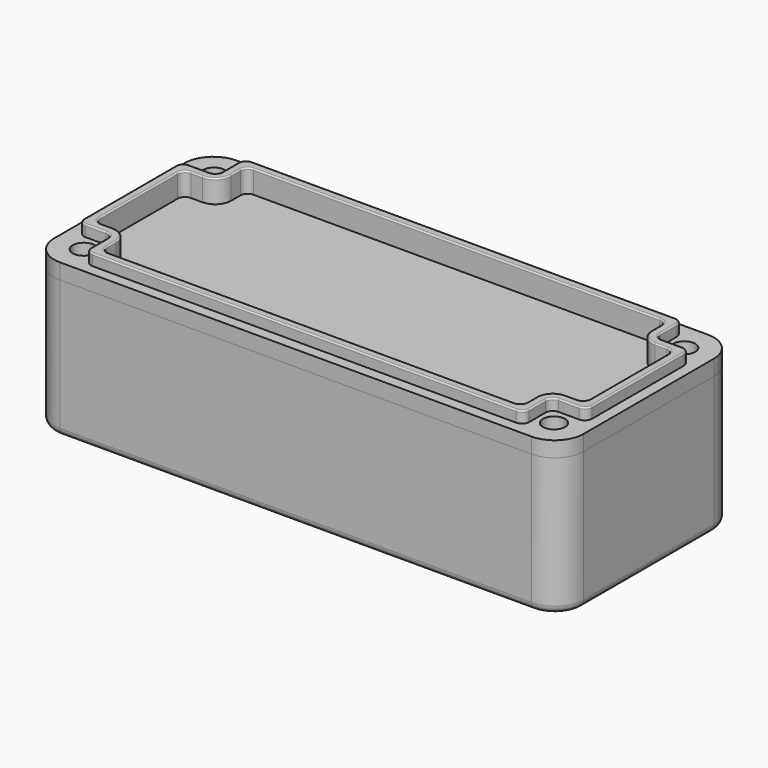
from build123d import *

# Parameters (mm, degrees)
F0_R     = 1.9431
F1_DEPTH = 26.924
F2_DEPTH = 25.4
F3_DEPTH = 3.9878
F4_DEPTH = 2.032
F5_DEPTH = 1.9812
F6_R     = 1.27
F7_SIZE  = 1.778
F8_SIZE  = 1.778
F9_R     = 0.254
F10_R    = 1.27


with BuildPart() as f1:
    # F0 (on Top) → F1 (new body)
    with BuildSketch(Plane.XY):
        with BuildLine():
            ThreePointArc((46.482, 14.2875), (44.9941024484, 17.8796024484), (41.402, 19.3675))
            Line((41.402, 19.3675), (38.4556, 19.3675))
            Line((38.4556, 19.3675), (-41.402, 19.3675))
            ThreePointArc((-41.402, 19.3675), (-44.9941024484, 17.8796024484), (-46.482, 14.2875))
            Line((-46.482, 14.2875), (-46.482, -11.3411))
            Line((-46.482, -11.3411), (-46.482, -14.2875))
            ThreePointArc((-46.482, -14.2875), (-44.9941024484, -17.8796024484), (-41.402, -19.3675))
            Line((-41.402, -19.3675), (-38.4556, -19.3675))
            Line((-38.4556, -19.3675), (38.4556, -19.3675))
            Line((38.4556, -19.3675), (41.402, -19.3675))
            ThreePointArc((41.402, -19.3675), (44.9941024484, -17.8796024484), (46.482, -14.2875))
            Line((46.482, -14.2875), (46.482, -11.3411))
            Line((46.482, -11.3411), (46.482, 11.3411))
            Line((46.482, 11.3411), (46.482, 14.2875))
        make_face()
        with Locations((-41.275, -14.2875)):
            Circle(F0_R, mode=Mode.SUBTRACT)
        with Locations((41.275, -14.2875)):
            Circle(F0_R, mode=Mode.SUBTRACT)
        with Locations((-41.275, 14.2875)):
            Circle(F0_R, mode=Mode.SUBTRACT)
        with BuildLine():
            ThreePointArc((38.4556, -16.1925), (38.0836256121, -17.0905256121), (37.1856, -17.4625))
            Line((37.1856, -17.4625), (-37.1856, -17.4625))
            ThreePointArc((-37.1856, -17.4625), (-38.0836256121, -17.0905256121), (-38.4556, -16.1925))
            Line((-38.4556, -16.1925), (-38.4556, -12.6111))
            ThreePointArc((-38.4556, -12.6111), (-38.8275743879, -11.7130743879), (-39.7256, -11.3411))
            Line((-39.7256, -11.3411), (-43.307, -11.3411))
            ThreePointArc((-43.307, -11.3411), (-44.2050256121, -10.9691256121), (-44.577, -10.0711))
            Line((-44.577, -10.0711), (-44.577, 10.0711))
            ThreePointArc((-44.577, 10.0711), (-44.2050256121, 10.9691256121), (-43.307, 11.3411))
            Line((-43.307, 11.3411), (-39.7256, 11.3411))
            ThreePointArc((-39.7256, 11.3411), (-38.8275743879, 11.7130743879), (-38.4556, 12.6111))
            Line((-38.4556, 12.6111), (-38.4556, 16.1925))
            ThreePointArc((-38.4556, 16.1925), (-38.0836256121, 17.0905256121), (-37.1856, 17.4625))
            Line((-37.1856, 17.4625), (37.1856, 17.4625))
            ThreePointArc((37.1856, 17.4625), (38.0836256121, 17.0905256121), (38.4556, 16.1925))
            Line((38.4556, 16.1925), (38.4556, 12.6111))
            ThreePointArc((38.4556, 12.6111), (38.8275743879, 11.7130743879), (39.7256, 11.3411))
            Line((39.7256, 11.3411), (43.307, 11.3411))
            ThreePointArc((43.307, 11.3411), (44.2050256121, 10.9691256121), (44.577, 10.0711))
            Line((44.577, 10.0711), (44.577, -10.0711))
            ThreePointArc((44.577, -10.0711), (44.2050256121, -10.9691256121), (43.307, -11.3411))
            Line((43.307, -11.3411), (39.7256, -11.3411))
            ThreePointArc((39.7256, -11.3411), (38.8275743879, -11.7130743879), (38.4556, -12.6111))
            Line((38.4556, -12.6111), (38.4556, -16.1925))
        make_face(mode=Mode.SUBTRACT)
        with Locations((41.275, 14.2875)):
            Circle(F0_R, mode=Mode.SUBTRACT)
        with BuildLine():
            Line((-37.1856, -17.4625), (37.1856, -17.4625))
            ThreePointArc((37.1856, -17.4625), (38.0836256121, -17.0905256121), (38.4556, -16.1925))
            Line((38.4556, -16.1925), (38.4556, -12.6111))
            ThreePointArc((38.4556, -12.6111), (38.8275743879, -11.7130743879), (39.7256, -11.3411))
            Line((39.7256, -11.3411), (43.307, -11.3411))
            ThreePointArc((43.307, -11.3411), (44.2050256121, -10.9691256121), (44.577, -10.0711))
            Line((44.577, -10.0711), (44.577, 10.0711))
            ThreePointArc((44.577, 10.0711), (44.2050256121, 10.9691256121), (43.307, 11.3411))
            Line((43.307, 11.3411), (39.7256, 11.3411))
            ThreePointArc((39.7256, 11.3411), (38.8275743879, 11.7130743879), (38.4556, 12.6111))
            Line((38.4556, 12.6111), (38.4556, 16.1925))
            ThreePointArc((38.4556, 16.1925), (38.0836256121, 17.0905256121), (37.1856, 17.4625))
            Line((37.1856, 17.4625), (-37.1856, 17.4625))
            ThreePointArc((-37.1856, 17.4625), (-38.0836256121, 17.0905256121), (-38.4556, 16.1925))
            Line((-38.4556, 16.1925), (-38.4556, 12.6111))
            ThreePointArc((-38.4556, 12.6111), (-38.8275743879, 11.7130743879), (-39.7256, 11.3411))
            Line((-39.7256, 11.3411), (-43.307, 11.3411))
            ThreePointArc((-43.307, 11.3411), (-44.2050256121, 10.9691256121), (-44.577, 10.0711))
            Line((-44.577, 10.0711), (-44.577, -10.0711))
            ThreePointArc((-44.577, -10.0711), (-44.2050256121, -10.9691256121), (-43.307, -11.3411))
            Line((-43.307, -11.3411), (-39.7256, -11.3411))
            ThreePointArc((-39.7256, -11.3411), (-38.8275743879, -11.7130743879), (-38.4556, -12.6111))
            Line((-38.4556, -12.6111), (-38.4556, -16.1925))
            ThreePointArc((-38.4556, -16.1925), (-38.0836256121, -17.0905256121), (-37.1856, -17.4625))
        make_face()
        with BuildLine():
            Line((-35.6616, 15.9385), (35.6616, 15.9385))
            ThreePointArc((35.6616, 15.9385), (36.5596256121, 15.5665256121), (36.9316, 14.6685))
            Line((36.9316, 14.6685), (36.9316, 12.6111))
            ThreePointArc((36.9316, 12.6111), (37.7499436534, 10.6354436534), (39.7256, 9.8171))
            Line((39.7256, 9.8171), (41.783, 9.8171))
            ThreePointArc((41.783, 9.8171), (42.6810256121, 9.4451256121), (43.053, 8.5471))
            Line((43.053, 8.5471), (43.053, -8.5471))
            ThreePointArc((43.053, -8.5471), (42.6810256121, -9.4451256121), (41.783, -9.8171))
            Line((41.783, -9.8171), (39.7256, -9.8171))
            ThreePointArc((39.7256, -9.8171), (37.7499436534, -10.6354436534), (36.9316, -12.6111))
            Line((36.9316, -12.6111), (36.9316, -14.6685))
            ThreePointArc((36.9316, -14.6685), (36.5596256121, -15.5665256121), (35.6616, -15.9385))
            Line((35.6616, -15.9385), (-35.6616, -15.9385))
            ThreePointArc((-35.6616, -15.9385), (-36.5596256121, -15.5665256121), (-36.9316, -14.6685))
            Line((-36.9316, -14.6685), (-36.9316, -12.6111))
            ThreePointArc((-36.9316, -12.6111), (-37.7499436534, -10.6354436534), (-39.7256, -9.8171))
            Line((-39.7256, -9.8171), (-41.783, -9.8171))
            ThreePointArc((-41.783, -9.8171), (-42.6810256121, -9.4451256121), (-43.053, -8.5471))
            Line((-43.053, -8.5471), (-43.053, 8.5471))
            ThreePointArc((-43.053, 8.5471), (-42.6810256121, 9.4451256121), (-41.783, 9.8171))
            Line((-41.783, 9.8171), (-39.7256, 9.8171))
            ThreePointArc((-39.7256, 9.8171), (-37.7499436534, 10.6354436534), (-36.9316, 12.6111))
            Line((-36.9316, 12.6111), (-36.9316, 14.6685))
            ThreePointArc((-36.9316, 14.6685), (-36.5596256121, 15.5665256121), (-35.6616, 15.9385))
        make_face(mode=Mode.SUBTRACT)
        with Locations((41.275, 14.2875)):
            Circle(F0_R)
        with Locations((41.275, -14.2875)):
            Circle(F0_R)
        with Locations((-41.275, -14.2875)):
            Circle(F0_R)
        with Locations((-41.275, 14.2875)):
            Circle(F0_R)
        with BuildLine():
            ThreePointArc((36.9316, 14.6685), (36.5596256121, 15.5665256121), (35.6616, 15.9385))
            Line((35.6616, 15.9385), (-35.6616, 15.9385))
            ThreePointArc((-35.6616, 15.9385), (-36.5596256121, 15.5665256121), (-36.9316, 14.6685))
            Line((-36.9316, 14.6685), (-36.9316, 12.6111))
            ThreePointArc((-36.9316, 12.6111), (-37.7499436534, 10.6354436534), (-39.7256, 9.8171))
            Line((-39.7256, 9.8171), (-41.783, 9.8171))
            ThreePointArc((-41.783, 9.8171), (-42.6810256121, 9.4451256121), (-43.053, 8.5471))
            Line((-43.053, 8.5471), (-43.053, -8.5471))
            ThreePointArc((-43.053, -8.5471), (-42.6810256121, -9.4451256121), (-41.783, -9.8171))
            Line((-41.783, -9.8171), (-39.7256, -9.8171))
            ThreePointArc((-39.7256, -9.8171), (-37.7499436534, -10.6354436534), (-36.9316, -12.6111))
            Line((-36.9316, -12.6111), (-36.9316, -14.6685))
            ThreePointArc((-36.9316, -14.6685), (-36.5596256121, -15.5665256121), (-35.6616, -15.9385))
            Line((-35.6616, -15.9385), (35.6616, -15.9385))
            ThreePointArc((35.6616, -15.9385), (36.5596256121, -15.5665256121), (36.9316, -14.6685))
            Line((36.9316, -14.6685), (36.9316, -12.6111))
            ThreePointArc((36.9316, -12.6111), (37.7499436534, -10.6354436534), (39.7256, -9.8171))
            Line((39.7256, -9.8171), (41.783, -9.8171))
            ThreePointArc((41.783, -9.8171), (42.6810256121, -9.4451256121), (43.053, -8.5471))
            Line((43.053, -8.5471), (43.053, 8.5471))
            ThreePointArc((43.053, 8.5471), (42.6810256121, 9.4451256121), (41.783, 9.8171))
            Line((41.783, 9.8171), (39.7256, 9.8171))
            ThreePointArc((39.7256, 9.8171), (37.7499436534, 10.6354436534), (36.9316, 12.6111))
            Line((36.9316, 12.6111), (36.9316, 14.6685))
        make_face()
    extrude(amount=-F1_DEPTH)

    # F0 (on Top) → F2 (cut)
    with BuildSketch(Plane.XY):
        with Locations((-41.275, 14.2875)):
            Circle(F0_R)
        with Locations((-41.275, -14.2875)):
            Circle(F0_R)
        with BuildLine():
            Line((-37.1856, -17.4625), (37.1856, -17.4625))
            ThreePointArc((37.1856, -17.4625), (38.0836256121, -17.0905256121), (38.4556, -16.1925))
            Line((38.4556, -16.1925), (38.4556, -12.6111))
            ThreePointArc((38.4556, -12.6111), (38.8275743879, -11.7130743879), (39.7256, -11.3411))
            Line((39.7256, -11.3411), (43.307, -11.3411))
            ThreePointArc((43.307, -11.3411), (44.2050256121, -10.9691256121), (44.577, -10.0711))
            Line((44.577, -10.0711), (44.577, 10.0711))
            ThreePointArc((44.577, 10.0711), (44.2050256121, 10.9691256121), (43.307, 11.3411))
            Line((43.307, 11.3411), (39.7256, 11.3411))
            ThreePointArc((39.7256, 11.3411), (38.8275743879, 11.7130743879), (38.4556, 12.6111))
            Line((38.4556, 12.6111), (38.4556, 16.1925))
            ThreePointArc((38.4556, 16.1925), (38.0836256121, 17.0905256121), (37.1856, 17.4625))
            Line((37.1856, 17.4625), (-37.1856, 17.4625))
            ThreePointArc((-37.1856, 17.4625), (-38.0836256121, 17.0905256121), (-38.4556, 16.1925))
            Line((-38.4556, 16.1925), (-38.4556, 12.6111))
            ThreePointArc((-38.4556, 12.6111), (-38.8275743879, 11.7130743879), (-39.7256, 11.3411))
            Line((-39.7256, 11.3411), (-43.307, 11.3411))
            ThreePointArc((-43.307, 11.3411), (-44.2050256121, 10.9691256121), (-44.577, 10.0711))
            Line((-44.577, 10.0711), (-44.577, -10.0711))
            ThreePointArc((-44.577, -10.0711), (-44.2050256121, -10.9691256121), (-43.307, -11.3411))
            Line((-43.307, -11.3411), (-39.7256, -11.3411))
            ThreePointArc((-39.7256, -11.3411), (-38.8275743879, -11.7130743879), (-38.4556, -12.6111))
            Line((-38.4556, -12.6111), (-38.4556, -16.1925))
            ThreePointArc((-38.4556, -16.1925), (-38.0836256121, -17.0905256121), (-37.1856, -17.4625))
        make_face()
        with BuildLine():
            Line((-35.6616, 15.9385), (35.6616, 15.9385))
            ThreePointArc((35.6616, 15.9385), (36.5596256121, 15.5665256121), (36.9316, 14.6685))
            Line((36.9316, 14.6685), (36.9316, 12.6111))
            ThreePointArc((36.9316, 12.6111), (37.7499436534, 10.6354436534), (39.7256, 9.8171))
            Line((39.7256, 9.8171), (41.783, 9.8171))
            ThreePointArc((41.783, 9.8171), (42.6810256121, 9.4451256121), (43.053, 8.5471))
            Line((43.053, 8.5471), (43.053, -8.5471))
            ThreePointArc((43.053, -8.5471), (42.6810256121, -9.4451256121), (41.783, -9.8171))
            Line((41.783, -9.8171), (39.7256, -9.8171))
            ThreePointArc((39.7256, -9.8171), (37.7499436534, -10.6354436534), (36.9316, -12.6111))
            Line((36.9316, -12.6111), (36.9316, -14.6685))
            ThreePointArc((36.9316, -14.6685), (36.5596256121, -15.5665256121), (35.6616, -15.9385))
            Line((35.6616, -15.9385), (-35.6616, -15.9385))
            ThreePointArc((-35.6616, -15.9385), (-36.5596256121, -15.5665256121), (-36.9316, -14.6685))
            Line((-36.9316, -14.6685), (-36.9316, -12.6111))
            ThreePointArc((-36.9316, -12.6111), (-37.7499436534, -10.6354436534), (-39.7256, -9.8171))
            Line((-39.7256, -9.8171), (-41.783, -9.8171))
            ThreePointArc((-41.783, -9.8171), (-42.6810256121, -9.4451256121), (-43.053, -8.5471))
            Line((-43.053, -8.5471), (-43.053, 8.5471))
            ThreePointArc((-43.053, 8.5471), (-42.6810256121, 9.4451256121), (-41.783, 9.8171))
            Line((-41.783, 9.8171), (-39.7256, 9.8171))
            ThreePointArc((-39.7256, 9.8171), (-37.7499436534, 10.6354436534), (-36.9316, 12.6111))
            Line((-36.9316, 12.6111), (-36.9316, 14.6685))
            ThreePointArc((-36.9316, 14.6685), (-36.5596256121, 15.5665256121), (-35.6616, 15.9385))
        make_face(mode=Mode.SUBTRACT)
        with Locations((41.275, 14.2875)):
            Circle(F0_R)
        with Locations((41.275, -14.2875)):
            Circle(F0_R)
        with BuildLine():
            ThreePointArc((36.9316, 14.6685), (36.5596256121, 15.5665256121), (35.6616, 15.9385))
            Line((35.6616, 15.9385), (-35.6616, 15.9385))
            ThreePointArc((-35.6616, 15.9385), (-36.5596256121, 15.5665256121), (-36.9316, 14.6685))
            Line((-36.9316, 14.6685), (-36.9316, 12.6111))
            ThreePointArc((-36.9316, 12.6111), (-37.7499436534, 10.6354436534), (-39.7256, 9.8171))
            Line((-39.7256, 9.8171), (-41.783, 9.8171))
            ThreePointArc((-41.783, 9.8171), (-42.6810256121, 9.4451256121), (-43.053, 8.5471))
            Line((-43.053, 8.5471), (-43.053, -8.5471))
            ThreePointArc((-43.053, -8.5471), (-42.6810256121, -9.4451256121), (-41.783, -9.8171))
            Line((-41.783, -9.8171), (-39.7256, -9.8171))
            ThreePointArc((-39.7256, -9.8171), (-37.7499436534, -10.6354436534), (-36.9316, -12.6111))
            Line((-36.9316, -12.6111), (-36.9316, -14.6685))
            ThreePointArc((-36.9316, -14.6685), (-36.5596256121, -15.5665256121), (-35.6616, -15.9385))
            Line((-35.6616, -15.9385), (35.6616, -15.9385))
            ThreePointArc((35.6616, -15.9385), (36.5596256121, -15.5665256121), (36.9316, -14.6685))
            Line((36.9316, -14.6685), (36.9316, -12.6111))
            ThreePointArc((36.9316, -12.6111), (37.7499436534, -10.6354436534), (39.7256, -9.8171))
            Line((39.7256, -9.8171), (41.783, -9.8171))
            ThreePointArc((41.783, -9.8171), (42.6810256121, -9.4451256121), (43.053, -8.5471))
            Line((43.053, -8.5471), (43.053, 8.5471))
            ThreePointArc((43.053, 8.5471), (42.6810256121, 9.4451256121), (41.783, 9.8171))
            Line((41.783, 9.8171), (39.7256, 9.8171))
            ThreePointArc((39.7256, 9.8171), (37.7499436534, 10.6354436534), (36.9316, 12.6111))
            Line((36.9316, 12.6111), (36.9316, 14.6685))
        make_face()
    extrude(amount=-F2_DEPTH, mode=Mode.SUBTRACT)

    # F10
    f10_edges = [f1.edges().sort_by_distance(p)[0] for p in [
        (0, 19.3675, -26.924),
        (44.994102, -17.879602, -26.924),
        (0, -19.3675, -26.924),
        (46.482, 0, -26.924),
        (44.994102, 17.879602, -26.924),
        (-44.994102, 17.879602, -26.924),
        (-46.482, 0, -26.924),
        (-44.994102, -17.879602, -26.924),
    ]]
    fillet(f10_edges, radius=F10_R)


with BuildPart() as f3:
    # F0 (on Top) → F3 (new body)
    with BuildSketch(Plane.XY):
        with BuildLine():
            ThreePointArc((46.482, 14.2875), (44.9941024484, 17.8796024484), (41.402, 19.3675))
            Line((41.402, 19.3675), (38.4556, 19.3675))
            Line((38.4556, 19.3675), (-41.402, 19.3675))
            ThreePointArc((-41.402, 19.3675), (-44.9941024484, 17.8796024484), (-46.482, 14.2875))
            Line((-46.482, 14.2875), (-46.482, -11.3411))
            Line((-46.482, -11.3411), (-46.482, -14.2875))
            ThreePointArc((-46.482, -14.2875), (-44.9941024484, -17.8796024484), (-41.402, -19.3675))
            Line((-41.402, -19.3675), (-38.4556, -19.3675))
            Line((-38.4556, -19.3675), (38.4556, -19.3675))
            Line((38.4556, -19.3675), (41.402, -19.3675))
            ThreePointArc((41.402, -19.3675), (44.9941024484, -17.8796024484), (46.482, -14.2875))
            Line((46.482, -14.2875), (46.482, -11.3411))
            Line((46.482, -11.3411), (46.482, 11.3411))
            Line((46.482, 11.3411), (46.482, 14.2875))
        make_face()
        with Locations((-41.275, -14.2875)):
            Circle(F0_R, mode=Mode.SUBTRACT)
        with Locations((41.275, -14.2875)):
            Circle(F0_R, mode=Mode.SUBTRACT)
        with Locations((-41.275, 14.2875)):
            Circle(F0_R, mode=Mode.SUBTRACT)
        with BuildLine():
            ThreePointArc((38.4556, -16.1925), (38.0836256121, -17.0905256121), (37.1856, -17.4625))
            Line((37.1856, -17.4625), (-37.1856, -17.4625))
            ThreePointArc((-37.1856, -17.4625), (-38.0836256121, -17.0905256121), (-38.4556, -16.1925))
            Line((-38.4556, -16.1925), (-38.4556, -12.6111))
            ThreePointArc((-38.4556, -12.6111), (-38.8275743879, -11.7130743879), (-39.7256, -11.3411))
            Line((-39.7256, -11.3411), (-43.307, -11.3411))
            ThreePointArc((-43.307, -11.3411), (-44.2050256121, -10.9691256121), (-44.577, -10.0711))
            Line((-44.577, -10.0711), (-44.577, 10.0711))
            ThreePointArc((-44.577, 10.0711), (-44.2050256121, 10.9691256121), (-43.307, 11.3411))
            Line((-43.307, 11.3411), (-39.7256, 11.3411))
            ThreePointArc((-39.7256, 11.3411), (-38.8275743879, 11.7130743879), (-38.4556, 12.6111))
            Line((-38.4556, 12.6111), (-38.4556, 16.1925))
            ThreePointArc((-38.4556, 16.1925), (-38.0836256121, 17.0905256121), (-37.1856, 17.4625))
            Line((-37.1856, 17.4625), (37.1856, 17.4625))
            ThreePointArc((37.1856, 17.4625), (38.0836256121, 17.0905256121), (38.4556, 16.1925))
            Line((38.4556, 16.1925), (38.4556, 12.6111))
            ThreePointArc((38.4556, 12.6111), (38.8275743879, 11.7130743879), (39.7256, 11.3411))
            Line((39.7256, 11.3411), (43.307, 11.3411))
            ThreePointArc((43.307, 11.3411), (44.2050256121, 10.9691256121), (44.577, 10.0711))
            Line((44.577, 10.0711), (44.577, -10.0711))
            ThreePointArc((44.577, -10.0711), (44.2050256121, -10.9691256121), (43.307, -11.3411))
            Line((43.307, -11.3411), (39.7256, -11.3411))
            ThreePointArc((39.7256, -11.3411), (38.8275743879, -11.7130743879), (38.4556, -12.6111))
            Line((38.4556, -12.6111), (38.4556, -16.1925))
        make_face(mode=Mode.SUBTRACT)
        with Locations((41.275, 14.2875)):
            Circle(F0_R, mode=Mode.SUBTRACT)
        with BuildLine():
            Line((-37.1856, -17.4625), (37.1856, -17.4625))
            ThreePointArc((37.1856, -17.4625), (38.0836256121, -17.0905256121), (38.4556, -16.1925))
            Line((38.4556, -16.1925), (38.4556, -12.6111))
            ThreePointArc((38.4556, -12.6111), (38.8275743879, -11.7130743879), (39.7256, -11.3411))
            Line((39.7256, -11.3411), (43.307, -11.3411))
            ThreePointArc((43.307, -11.3411), (44.2050256121, -10.9691256121), (44.577, -10.0711))
            Line((44.577, -10.0711), (44.577, 10.0711))
            ThreePointArc((44.577, 10.0711), (44.2050256121, 10.9691256121), (43.307, 11.3411))
            Line((43.307, 11.3411), (39.7256, 11.3411))
            ThreePointArc((39.7256, 11.3411), (38.8275743879, 11.7130743879), (38.4556, 12.6111))
            Line((38.4556, 12.6111), (38.4556, 16.1925))
            ThreePointArc((38.4556, 16.1925), (38.0836256121, 17.0905256121), (37.1856, 17.4625))
            Line((37.1856, 17.4625), (-37.1856, 17.4625))
            ThreePointArc((-37.1856, 17.4625), (-38.0836256121, 17.0905256121), (-38.4556, 16.1925))
            Line((-38.4556, 16.1925), (-38.4556, 12.6111))
            ThreePointArc((-38.4556, 12.6111), (-38.8275743879, 11.7130743879), (-39.7256, 11.3411))
            Line((-39.7256, 11.3411), (-43.307, 11.3411))
            ThreePointArc((-43.307, 11.3411), (-44.2050256121, 10.9691256121), (-44.577, 10.0711))
            Line((-44.577, 10.0711), (-44.577, -10.0711))
            ThreePointArc((-44.577, -10.0711), (-44.2050256121, -10.9691256121), (-43.307, -11.3411))
            Line((-43.307, -11.3411), (-39.7256, -11.3411))
            ThreePointArc((-39.7256, -11.3411), (-38.8275743879, -11.7130743879), (-38.4556, -12.6111))
            Line((-38.4556, -12.6111), (-38.4556, -16.1925))
            ThreePointArc((-38.4556, -16.1925), (-38.0836256121, -17.0905256121), (-37.1856, -17.4625))
        make_face()
        with BuildLine():
            Line((-35.6616, 15.9385), (35.6616, 15.9385))
            ThreePointArc((35.6616, 15.9385), (36.5596256121, 15.5665256121), (36.9316, 14.6685))
            Line((36.9316, 14.6685), (36.9316, 12.6111))
            ThreePointArc((36.9316, 12.6111), (37.7499436534, 10.6354436534), (39.7256, 9.8171))
            Line((39.7256, 9.8171), (41.783, 9.8171))
            ThreePointArc((41.783, 9.8171), (42.6810256121, 9.4451256121), (43.053, 8.5471))
            Line((43.053, 8.5471), (43.053, -8.5471))
            ThreePointArc((43.053, -8.5471), (42.6810256121, -9.4451256121), (41.783, -9.8171))
            Line((41.783, -9.8171), (39.7256, -9.8171))
            ThreePointArc((39.7256, -9.8171), (37.7499436534, -10.6354436534), (36.9316, -12.6111))
            Line((36.9316, -12.6111), (36.9316, -14.6685))
            ThreePointArc((36.9316, -14.6685), (36.5596256121, -15.5665256121), (35.6616, -15.9385))
            Line((35.6616, -15.9385), (-35.6616, -15.9385))
            ThreePointArc((-35.6616, -15.9385), (-36.5596256121, -15.5665256121), (-36.9316, -14.6685))
            Line((-36.9316, -14.6685), (-36.9316, -12.6111))
            ThreePointArc((-36.9316, -12.6111), (-37.7499436534, -10.6354436534), (-39.7256, -9.8171))
            Line((-39.7256, -9.8171), (-41.783, -9.8171))
            ThreePointArc((-41.783, -9.8171), (-42.6810256121, -9.4451256121), (-43.053, -8.5471))
            Line((-43.053, -8.5471), (-43.053, 8.5471))
            ThreePointArc((-43.053, 8.5471), (-42.6810256121, 9.4451256121), (-41.783, 9.8171))
            Line((-41.783, 9.8171), (-39.7256, 9.8171))
            ThreePointArc((-39.7256, 9.8171), (-37.7499436534, 10.6354436534), (-36.9316, 12.6111))
            Line((-36.9316, 12.6111), (-36.9316, 14.6685))
            ThreePointArc((-36.9316, 14.6685), (-36.5596256121, 15.5665256121), (-35.6616, 15.9385))
        make_face(mode=Mode.SUBTRACT)
        with BuildLine():
            ThreePointArc((36.9316, 14.6685), (36.5596256121, 15.5665256121), (35.6616, 15.9385))
            Line((35.6616, 15.9385), (-35.6616, 15.9385))
            ThreePointArc((-35.6616, 15.9385), (-36.5596256121, 15.5665256121), (-36.9316, 14.6685))
            Line((-36.9316, 14.6685), (-36.9316, 12.6111))
            ThreePointArc((-36.9316, 12.6111), (-37.7499436534, 10.6354436534), (-39.7256, 9.8171))
            Line((-39.7256, 9.8171), (-41.783, 9.8171))
            ThreePointArc((-41.783, 9.8171), (-42.6810256121, 9.4451256121), (-43.053, 8.5471))
            Line((-43.053, 8.5471), (-43.053, -8.5471))
            ThreePointArc((-43.053, -8.5471), (-42.6810256121, -9.4451256121), (-41.783, -9.8171))
            Line((-41.783, -9.8171), (-39.7256, -9.8171))
            ThreePointArc((-39.7256, -9.8171), (-37.7499436534, -10.6354436534), (-36.9316, -12.6111))
            Line((-36.9316, -12.6111), (-36.9316, -14.6685))
            ThreePointArc((-36.9316, -14.6685), (-36.5596256121, -15.5665256121), (-35.6616, -15.9385))
            Line((-35.6616, -15.9385), (35.6616, -15.9385))
            ThreePointArc((35.6616, -15.9385), (36.5596256121, -15.5665256121), (36.9316, -14.6685))
            Line((36.9316, -14.6685), (36.9316, -12.6111))
            ThreePointArc((36.9316, -12.6111), (37.7499436534, -10.6354436534), (39.7256, -9.8171))
            Line((39.7256, -9.8171), (41.783, -9.8171))
            ThreePointArc((41.783, -9.8171), (42.6810256121, -9.4451256121), (43.053, -8.5471))
            Line((43.053, -8.5471), (43.053, 8.5471))
            ThreePointArc((43.053, 8.5471), (42.6810256121, 9.4451256121), (41.783, 9.8171))
            Line((41.783, 9.8171), (39.7256, 9.8171))
            ThreePointArc((39.7256, 9.8171), (37.7499436534, 10.6354436534), (36.9316, 12.6111))
            Line((36.9316, 12.6111), (36.9316, 14.6685))
        make_face()
    extrude(amount=-F3_DEPTH)

    # F0 (on Top) → F4 (cut)
    with BuildSketch(Plane.XY):
        with BuildLine():
            ThreePointArc((36.9316, 14.6685), (36.5596256121, 15.5665256121), (35.6616, 15.9385))
            Line((35.6616, 15.9385), (-35.6616, 15.9385))
            ThreePointArc((-35.6616, 15.9385), (-36.5596256121, 15.5665256121), (-36.9316, 14.6685))
            Line((-36.9316, 14.6685), (-36.9316, 12.6111))
            ThreePointArc((-36.9316, 12.6111), (-37.7499436534, 10.6354436534), (-39.7256, 9.8171))
            Line((-39.7256, 9.8171), (-41.783, 9.8171))
            ThreePointArc((-41.783, 9.8171), (-42.6810256121, 9.4451256121), (-43.053, 8.5471))
            Line((-43.053, 8.5471), (-43.053, -8.5471))
            ThreePointArc((-43.053, -8.5471), (-42.6810256121, -9.4451256121), (-41.783, -9.8171))
            Line((-41.783, -9.8171), (-39.7256, -9.8171))
            ThreePointArc((-39.7256, -9.8171), (-37.7499436534, -10.6354436534), (-36.9316, -12.6111))
            Line((-36.9316, -12.6111), (-36.9316, -14.6685))
            ThreePointArc((-36.9316, -14.6685), (-36.5596256121, -15.5665256121), (-35.6616, -15.9385))
            Line((-35.6616, -15.9385), (35.6616, -15.9385))
            ThreePointArc((35.6616, -15.9385), (36.5596256121, -15.5665256121), (36.9316, -14.6685))
            Line((36.9316, -14.6685), (36.9316, -12.6111))
            ThreePointArc((36.9316, -12.6111), (37.7499436534, -10.6354436534), (39.7256, -9.8171))
            Line((39.7256, -9.8171), (41.783, -9.8171))
            ThreePointArc((41.783, -9.8171), (42.6810256121, -9.4451256121), (43.053, -8.5471))
            Line((43.053, -8.5471), (43.053, 8.5471))
            ThreePointArc((43.053, 8.5471), (42.6810256121, 9.4451256121), (41.783, 9.8171))
            Line((41.783, 9.8171), (39.7256, 9.8171))
            ThreePointArc((39.7256, 9.8171), (37.7499436534, 10.6354436534), (36.9316, 12.6111))
            Line((36.9316, 12.6111), (36.9316, 14.6685))
        make_face()
    extrude(amount=-F4_DEPTH, mode=Mode.SUBTRACT)

    # F0 (on Top) → F5 (join)
    with BuildSketch(Plane.XY):
        with BuildLine():
            Line((-37.1856, -17.4625), (37.1856, -17.4625))
            ThreePointArc((37.1856, -17.4625), (38.0836256121, -17.0905256121), (38.4556, -16.1925))
            Line((38.4556, -16.1925), (38.4556, -12.6111))
            ThreePointArc((38.4556, -12.6111), (38.8275743879, -11.7130743879), (39.7256, -11.3411))
            Line((39.7256, -11.3411), (43.307, -11.3411))
            ThreePointArc((43.307, -11.3411), (44.2050256121, -10.9691256121), (44.577, -10.0711))
            Line((44.577, -10.0711), (44.577, 10.0711))
            ThreePointArc((44.577, 10.0711), (44.2050256121, 10.9691256121), (43.307, 11.3411))
            Line((43.307, 11.3411), (39.7256, 11.3411))
            ThreePointArc((39.7256, 11.3411), (38.8275743879, 11.7130743879), (38.4556, 12.6111))
            Line((38.4556, 12.6111), (38.4556, 16.1925))
            ThreePointArc((38.4556, 16.1925), (38.0836256121, 17.0905256121), (37.1856, 17.4625))
            Line((37.1856, 17.4625), (-37.1856, 17.4625))
            ThreePointArc((-37.1856, 17.4625), (-38.0836256121, 17.0905256121), (-38.4556, 16.1925))
            Line((-38.4556, 16.1925), (-38.4556, 12.6111))
            ThreePointArc((-38.4556, 12.6111), (-38.8275743879, 11.7130743879), (-39.7256, 11.3411))
            Line((-39.7256, 11.3411), (-43.307, 11.3411))
            ThreePointArc((-43.307, 11.3411), (-44.2050256121, 10.9691256121), (-44.577, 10.0711))
            Line((-44.577, 10.0711), (-44.577, -10.0711))
            ThreePointArc((-44.577, -10.0711), (-44.2050256121, -10.9691256121), (-43.307, -11.3411))
            Line((-43.307, -11.3411), (-39.7256, -11.3411))
            ThreePointArc((-39.7256, -11.3411), (-38.8275743879, -11.7130743879), (-38.4556, -12.6111))
            Line((-38.4556, -12.6111), (-38.4556, -16.1925))
            ThreePointArc((-38.4556, -16.1925), (-38.0836256121, -17.0905256121), (-37.1856, -17.4625))
        make_face()
        with BuildLine():
            Line((-35.6616, 15.9385), (35.6616, 15.9385))
            ThreePointArc((35.6616, 15.9385), (36.5596256121, 15.5665256121), (36.9316, 14.6685))
            Line((36.9316, 14.6685), (36.9316, 12.6111))
            ThreePointArc((36.9316, 12.6111), (37.7499436534, 10.6354436534), (39.7256, 9.8171))
            Line((39.7256, 9.8171), (41.783, 9.8171))
            ThreePointArc((41.783, 9.8171), (42.6810256121, 9.4451256121), (43.053, 8.5471))
            Line((43.053, 8.5471), (43.053, -8.5471))
            ThreePointArc((43.053, -8.5471), (42.6810256121, -9.4451256121), (41.783, -9.8171))
            Line((41.783, -9.8171), (39.7256, -9.8171))
            ThreePointArc((39.7256, -9.8171), (37.7499436534, -10.6354436534), (36.9316, -12.6111))
            Line((36.9316, -12.6111), (36.9316, -14.6685))
            ThreePointArc((36.9316, -14.6685), (36.5596256121, -15.5665256121), (35.6616, -15.9385))
            Line((35.6616, -15.9385), (-35.6616, -15.9385))
            ThreePointArc((-35.6616, -15.9385), (-36.5596256121, -15.5665256121), (-36.9316, -14.6685))
            Line((-36.9316, -14.6685), (-36.9316, -12.6111))
            ThreePointArc((-36.9316, -12.6111), (-37.7499436534, -10.6354436534), (-39.7256, -9.8171))
            Line((-39.7256, -9.8171), (-41.783, -9.8171))
            ThreePointArc((-41.783, -9.8171), (-42.6810256121, -9.4451256121), (-43.053, -8.5471))
            Line((-43.053, -8.5471), (-43.053, 8.5471))
            ThreePointArc((-43.053, 8.5471), (-42.6810256121, 9.4451256121), (-41.783, 9.8171))
            Line((-41.783, 9.8171), (-39.7256, 9.8171))
            ThreePointArc((-39.7256, 9.8171), (-37.7499436534, 10.6354436534), (-36.9316, 12.6111))
            Line((-36.9316, 12.6111), (-36.9316, 14.6685))
            ThreePointArc((-36.9316, 14.6685), (-36.5596256121, 15.5665256121), (-35.6616, 15.9385))
        make_face(mode=Mode.SUBTRACT)
    extrude(amount=F5_DEPTH)

    # F6
    f6_edges = [f3.edges().sort_by_distance(p)[0] for p in [
        (-46.482, 0, -3.9878),
    ]]
    fillet(f6_edges, radius=F6_R)

    # F7
    f7_edges = [f3.edges().sort_by_distance(p)[0] for p in [
        (-43.2181, 14.2875, -3.9878),
    ]]
    chamfer(f7_edges, length=F7_SIZE)

    # F8
    f8_edges = [f3.edges().sort_by_distance(p)[0] for p in [
        (-43.2181, -14.2875, -3.9878),
        (39.3319, 14.2875, -3.9878),
        (39.3319, -14.2875, -3.9878),
    ]]
    chamfer(f8_edges, length=F8_SIZE)

    # F9
    f9_edges = [f3.edges().sort_by_distance(p)[0] for p in [
        (0, -17.4625, 1.9812),
        (0, 15.9385, 1.9812),
        (-38.827574, -11.713074, 1.9812),
        (-38.4556, -14.4018, 1.9812),
        (-38.083626, -17.090526, 1.9812),
        (38.083626, -17.090526, 1.9812),
        (38.4556, -14.4018, 1.9812),
        (38.827574, -11.713074, 1.9812),
        (41.5163, -11.3411, 1.9812),
        (44.205026, -10.969126, 1.9812),
        (44.577, 0, 1.9812),
        (44.205026, 10.969126, 1.9812),
        (41.5163, 11.3411, 1.9812),
        (38.827574, 11.713074, 1.9812),
        (38.4556, 14.4018, 1.9812),
        (38.083626, 17.090526, 1.9812),
        (0, 17.4625, 1.9812),
        (-38.083626, 17.090526, 1.9812),
        (-38.4556, 14.4018, 1.9812),
        (-38.827574, 11.713074, 1.9812),
        (-41.5163, 11.3411, 1.9812),
        (-44.205026, 10.969126, 1.9812),
        (-44.577, 0, 1.9812),
        (-44.205026, -10.969126, 1.9812),
        (-41.5163, -11.3411, 1.9812),
        (-36.559626, -15.566526, 1.9812),
        (-36.9316, -13.6398, 1.9812),
        (-37.749944, -10.635444, 1.9812),
        (-40.7543, -9.8171, 1.9812),
        (-42.681026, -9.445126, 1.9812),
        (-43.053, 0, 1.9812),
        (-42.681026, 9.445126, 1.9812),
        (-40.7543, 9.8171, 1.9812),
        (-37.749944, 10.635444, 1.9812),
        (-36.9316, 13.6398, 1.9812),
        (-36.559626, 15.566526, 1.9812),
        (36.559626, 15.566526, 1.9812),
        (36.9316, 13.6398, 1.9812),
        (37.749944, 10.635444, 1.9812),
        (40.7543, 9.8171, 1.9812),
        (42.681026, 9.445126, 1.9812),
        (43.053, 0, 1.9812),
        (42.681026, -9.445126, 1.9812),
        (40.7543, -9.8171, 1.9812),
        (37.749944, -10.635444, 1.9812),
        (36.9316, -13.6398, 1.9812),
        (36.559626, -15.566526, 1.9812),
        (0, -15.9385, 1.9812),
    ]]
    fillet(f9_edges, radius=F9_R)


solid = Compound([f1.part, f3.part])
